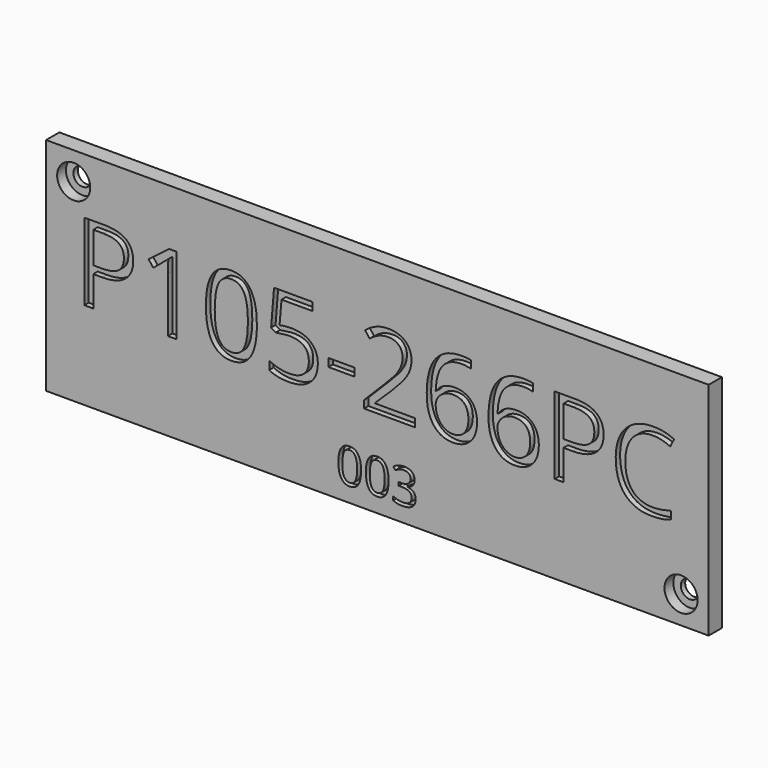
from build123d import *

# Parameters (mm, degrees)
F0_W           = 120
F0_H           = 40
F1_DEPTH       = 3
F3_D           = 3.3
F3_CBORE_D     = 6
F3_CBORE_DEPTH = 2
F4_TEXT_SIZE   = 19.5658819933
F5_DEPTH       = 1
F6_TEXT_SIZE   = 8.7138059363
F7_DEPTH       = 1


# Not quite as in the source:
# - Text() gives the source's letters only with a copy of the font that has no kerning and outlines rounded to 1/6400 em; it was checked with that copy


with BuildPart() as f1:
    # F0 (on Front) → F1 (new body)
    with BuildSketch(Plane.XZ):
        Rectangle(F0_W, F0_H)
    extrude(amount=F1_DEPTH)

    # F3 (through all)
    with Locations(Plane.XZ.offset(3)):
        with Locations((-55, 15), (55, -15)):
            CounterBoreHole(F3_D / 2, F3_CBORE_D / 2, F3_CBORE_DEPTH)

    # F4 (on face) → F5 (cut)
    with BuildSketch(Plane.XZ.offset(3)):
        with Locations((-55, -4.0874350352)):
            Text('P105-266PC', F4_TEXT_SIZE, font='Open Sans', text_align=(TextAlign.LEFT, TextAlign.BOTTOM))
    extrude(amount=-F5_DEPTH, mode=Mode.SUBTRACT)

    # F6 (on face) → F7 (cut)
    with BuildSketch(Plane.XZ.offset(3)):
        with Locations((-7.5, -17.2739402741)):
            Text('003', F6_TEXT_SIZE, font='Open Sans', text_align=(TextAlign.LEFT, TextAlign.BOTTOM))
    extrude(amount=-F7_DEPTH, mode=Mode.SUBTRACT)


solid = f1.part
